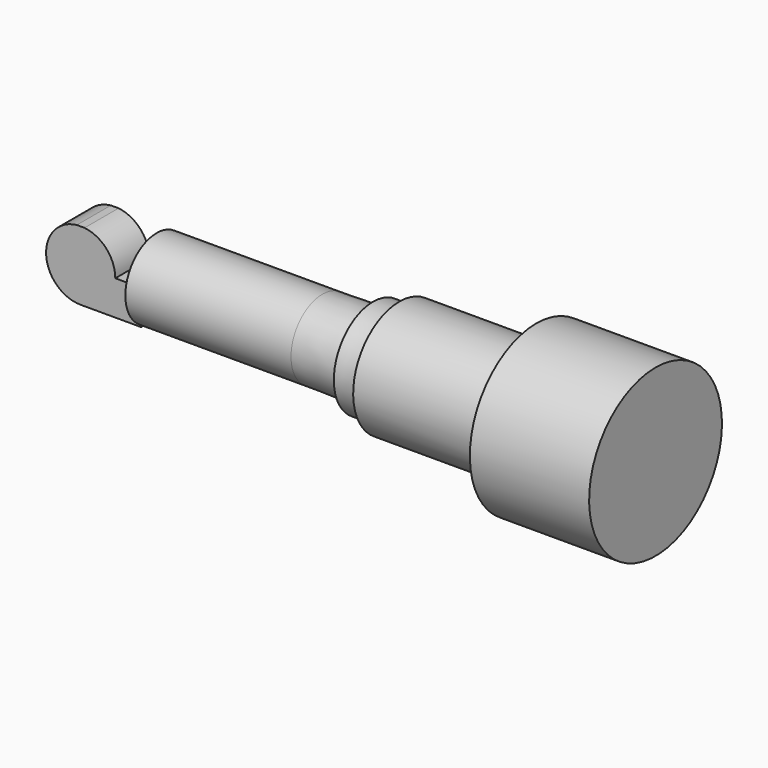
from build123d import *
from build123d import SkipClean  # not in build123d's __all__

# Parameters (mm, degrees)
F3_DEPTH = 12.7


with BuildPart() as f1:
    # F0 (on Front) → F1 (revolve)
    with BuildSketch(Plane.XZ):
        Polygon((30.2789051418, 45.5598932677), (30.4273499666, 40.2938460652), (61.5186302682, 40.8079418176), (154.2716920376, 40.8079418176), (154.7678885906, 16.2854908297), (199.0363299847, 16.2854908297), (199.0363299847, 36.9584394366), (199.0363299847, 65.8766925335), (127.791211009, 65.8766925335), (127.791211009, 50.7449842989), (45.9729901174, 50.7449842989), (46.0544126905, 45.8207420119), align=None)
    revolve(axis=Axis((-33.7930093709, 0, 16.2854908297), (1, 0, 0)))


with BuildPart() as f2:
    # F0 (on Front) → F2 (revolve)
    with BuildSketch(Plane.XZ):
        Polygon((-98.9724991263, 39.6781675518), (-98.4991628533, 16.2854908297), (30.9131441116, 16.2854908297), (30.4273499666, 40.2938460652), (0, 39.6781675518), align=None)
        Polygon((30.4273499666, 40.2938460652), (30.9131441116, 16.2854908297), (62.0148268213, 16.2854908297), (61.5186302682, 40.8079418176), align=None)
    revolve(axis=Axis((-33.7930093709, 0, 16.2854908297), (1, 0, 0)))

    # F0 (on Front) → F3 (join, symmetric)
    with BuildSketch(Plane.XZ):
        with BuildLine():
            Line((-131.8934512444, 36.8291237046), (-136.5107891798, 36.8291237046))
            ThreePointArc((-136.5107891798, 36.8291237046), (-154.8427145679, 15.1293469199), (-134.2021202121, -4.3874577771))
            ThreePointArc((-134.2021202121, -4.3874577771), (-119.5841380651, 1.6675086827), (-113.5291716052, 16.2854908297))
            ThreePointArc((-113.5291716052, 16.2854908297), (-118.7894987767, 30.0630778678), (-131.8934512444, 36.8291237046))
        make_face()
        with BuildLine():
            ThreePointArc((-113.5291716052, 16.2854908297), (-119.5841380651, 1.6675086827), (-134.2021202121, -4.3874577771))
            Line((-134.2021202121, -4.3874577771), (-98.0808585882, -4.3874577771))
            Line((-98.0808585882, -4.3874577771), (-98.4991628533, 16.2854908297))
            Line((-98.4991628533, 16.2854908297), (-113.5291716052, 16.2854908297))
        make_face()
    with SkipClean():  # cleaning this boolean's faces spoils the solid; the shape is the same uncleaned
        extrude(amount=F3_DEPTH, both=True)


solid = Compound([f1.part, f2.part])
